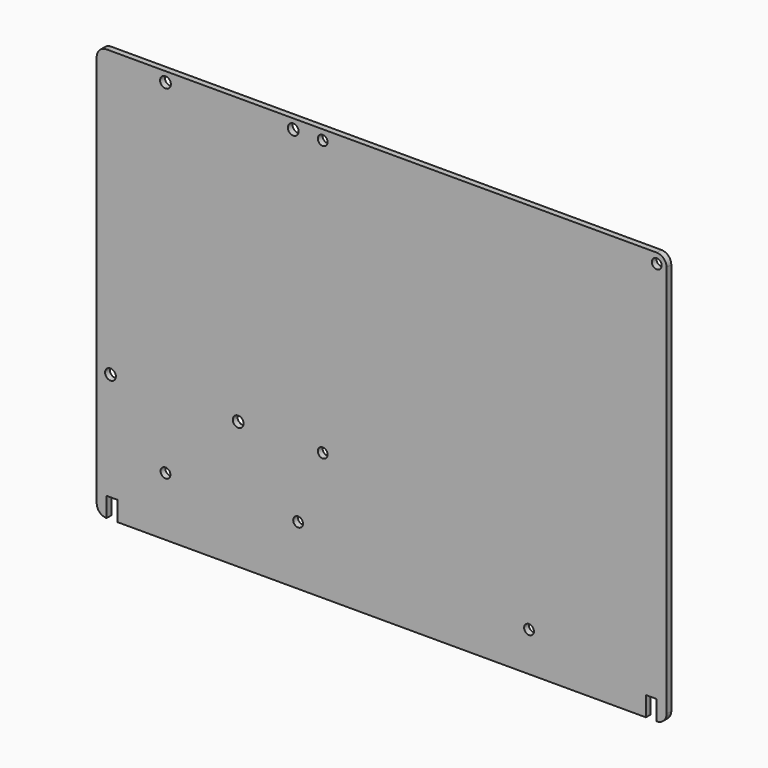
from build123d import *

# Parameters (mm, degrees)
F1_DEPTH = 3
F2_R     = 2.75
F3_DEPTH = 3
F4_R     = 2.5
F5_DEPTH = 3
F6_R     = 2.5
F7_DEPTH = 3
F8_R     = 4.99999


# Not quite as in the source:
# - a fillet or chamfer is up to 0.001 mm smaller than in the source, because OpenCascade refuses the exact size


with BuildPart() as f1:
    # F0 (on Front) → F1 (new body)
    with BuildSketch(Plane.XZ):
        Polygon((140, -105), (145, -105), (145, 105), (-145, 105), (-145, -105), (-140, -105), (-140, -95), (-134.5, -95), (-134.5, -105), (134.5, -105), (134.5, -95), (140, -95), align=None)
    extrude(amount=F1_DEPTH)

    # F2 (on face) → F3 (cut, through all)
    with BuildSketch(Plane.XZ.offset(3)):
        with Locations((-110, 100)):
            Circle(F2_R)
        with Locations((-138, -40)):
            Circle(F2_R)
        with Locations((-45, 100)):
            Circle(F2_R)
        with Locations((-73, -40)):
            Circle(F2_R)
    extrude(amount=-F3_DEPTH, mode=Mode.SUBTRACT)

    # F4 (on face) → F5 (cut, through all)
    with BuildSketch(Plane.XZ.offset(3)):
        with Locations((-30, 100)):
            Circle(F4_R)
        with Locations((140, 100)):
            Circle(F4_R)
        with Locations((75, -85)):
            Circle(F4_R)
        with Locations((-30, -40)):
            Circle(F4_R)
    extrude(amount=-F5_DEPTH, mode=Mode.SUBTRACT)

    # F6 (on face) → F7 (cut, through all)
    with BuildSketch(Plane.XZ.offset(3)):
        with Locations((-110, -75)):
            Circle(F6_R)
        with Locations((-42.5, -75)):
            Circle(F6_R)
    extrude(amount=-F7_DEPTH, mode=Mode.SUBTRACT)

    # F8 (radius 5 in the source; OpenCascade refuses exactly that, so slightly less here)
    f8_edges = [f1.edges().sort_by_distance(p)[0] for p in [
        (-145, -1.5, 105),
        (145, -1.5, 105),
        (145, -1.5, -105),
        (-145, -1.5, -105),
    ]]
    fillet(f8_edges, radius=F8_R)


solid = f1.part
